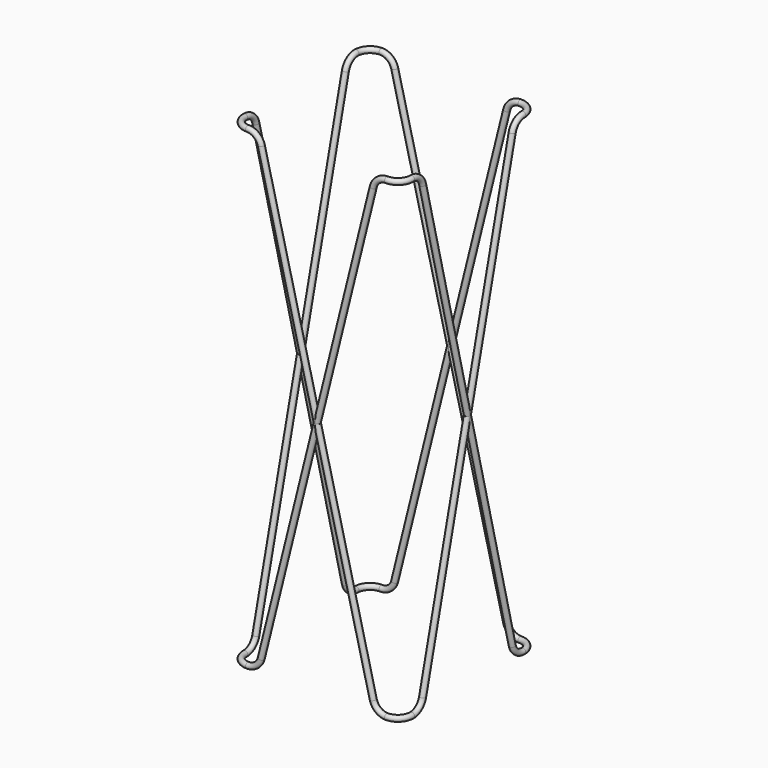
from build123d import *

# Parameters (mm, degrees)
F9_R              = 5
F10_COPIES1_COUNT = 2


# Not quite as in the source:
# - a feature of the source that left no trace in its solid (it failed there, or was rolled back) is left out
# - a pattern or mirror of a feature is missing from the dataset's text; its kind, count and spacing are read off the source's solid


with BuildPart() as f10:
    # F10: sweep along a path in F7, F2, F0, F5, F7
    with BuildLine(Plane.XY.offset(-850)) as f10_path:
        ThreePointArc((125, -150), (142.6776695297, -142.6776695297), (150, -125))
    with BuildLine(Plane.XZ.offset(150)) as f10_path_2:
        ThreePointArc((125, -850), (109.5971216154, -844.6914026283), (100.7356576076, -831.0201069976))
        Line((100.7356576076, -831.0201069976), (-100.7356576076, -18.9798930024))
        ThreePointArc((-100.7356576076, -18.9798930024), (-109.5971216154, -5.3085973717), (-125, 0))
    with BuildLine(Plane.XY) as f10_path_3:
        ThreePointArc((-150, -125), (-142.6776695297, -142.6776695297), (-125, -150))
    with BuildLine(Plane.YZ.offset(-150)) as f10_path_4:
        ThreePointArc((-125, 0), (-109.5971216154, -5.3085973717), (-100.7356576076, -18.9798930024))
        Line((-100.7356576076, -18.9798930024), (100.7356576076, -831.0201069976))
        ThreePointArc((100.7356576076, -831.0201069976), (109.5971216154, -844.6914026283), (125, -850))
    with BuildLine(Plane.XY.offset(-850)) as f10_path_5:
        ThreePointArc((-125, 150), (-142.6776695297, 142.6776695297), (-150, 125))
    # F9 (on plane+point) → F10 (sweep)
    with BuildSketch(Plane.XZ.offset(125)):
        with Locations((150, -850)):
            Circle(F9_R)
    sweep(path=f10_path.line + f10_path_2.line + f10_path_3.line + f10_path_4.line + f10_path_5.line)

    # F10_copies: F10 across plane


with BuildPart() as f10_1:
    add(f10.part)
    add(f10.part.mirror(Plane.XY.offset(-425)))

    # F10_copies1: F10 ×2 about axis
    f10_copies1_axis = Axis((0, 0, 0), (0, 0, 1))


with BuildPart() as f10_2:
    add(f10_1.part)
    for i in range(1, F10_COPIES1_COUNT):
        add(f10_1.part.rotate(f10_copies1_axis, i * 360 / F10_COPIES1_COUNT))


solid = f10_2.part
